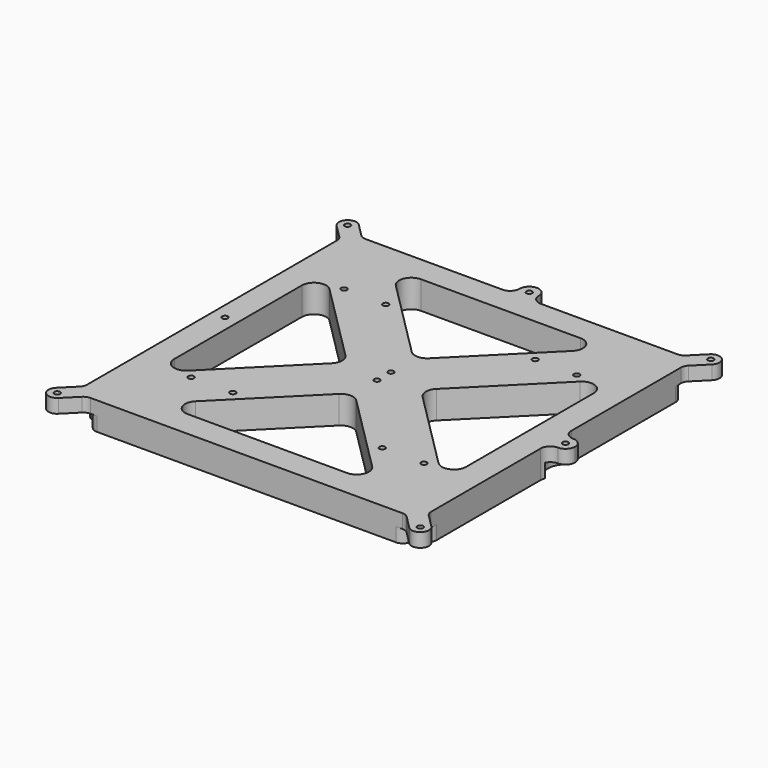
from build123d import *

# Parameters (mm, degrees)
F0_W         = 198
F0_H         = 198
F1_DEPTH     = 16
F2_W         = 11
F2_H         = 11
F3_DEPTH     = 16
F5_DEPTH     = 8
F6_R         = 5
F7_R         = 7
F8_T1_DEPTH  = 35.5
F8_T3_DEPTH  = 8
F8_T8_DEPTH  = 35.5
F8_S11_R     = 10
F8_T12_DEPTH = 20
F8_T16_DEPTH = 35.5
F8_S19_R     = 10
F8_T20_DEPTH = 20
F8_T24_DEPTH = 35.5
F8_S27_R     = 10
F8_T28_DEPTH = 20
F8_T32_DEPTH = 35.5
F8_S35_R     = 10
F8_T36_DEPTH = 20
F9_D         = 3.3
F10_D        = 3.3
F11_D        = 3.3


# Not quite as in the source:
# - a fillet or chamfer that OpenCascade refuses, or shapes differently, is made with other operations: its cross-section is extruded or revolved along the edge and cut away or added
# - ends of sketch curves that miss each other by under 0.0002 mm in the source are joined


with BuildPart() as f1:
    # F0 (on Top) → F1 (new body)
    with BuildSketch(Plane.XY):
        Rectangle(F0_W, F0_H)
        Polygon((-62.7867965644, -84), (0, -21.2132034356), (62.7867965644, -84), align=None, mode=Mode.SUBTRACT)
        Polygon((84, -62.7867965644), (21.2132034356, 0), (84, 62.7867965644), align=None, mode=Mode.SUBTRACT)
        Polygon((-84, 62.7867965644), (-21.2132034356, 0), (-84, -62.7867965644), align=None, mode=Mode.SUBTRACT)
        Polygon((62.7867965644, 84), (0, 21.2132034356), (-62.7867965644, 84), align=None, mode=Mode.SUBTRACT)
    extrude(amount=F1_DEPTH)

    # F2 (on face) → F3 (join, through all)
    with BuildSketch(Plane.XY.offset(16)):
        with BuildLine():
            Line((-99, -99), (-99, -91.9289296269))
            Line((-99, -91.9289296269), (-108.0355351865, -100.9644648135))
            ThreePointArc((-108.0355351865, -100.9644648135), (-108.0355351865, -108.0355351865), (-100.9644648135, -108.0355351865))
            Line((-100.9644648135, -108.0355351865), (-91.9289321881, -99))
            Line((-91.9289321881, -99), (-99, -99))
        make_face()
        with BuildLine():
            Line((99, -99), (91.9289321881, -99))
            Line((91.9289321881, -99), (100.9644660941, -108.0355339059))
            ThreePointArc((100.9644660941, -108.0355339059), (108.0355351865, -108.0355351865), (108.0355351865, -100.9644648135))
            Line((108.0355351865, -100.9644648135), (99, -91.9289296269))
            Line((99, -91.9289296269), (99, -99))
        make_face()
        with Locations((104.5, 0)):
            Rectangle(F2_W, F2_H)
        with BuildLine():
            Line((100.9644660941, 108.0355339059), (91.9289321881, 99))
            Line((91.9289321881, 99), (99, 99))
            Line((99, 99), (99, 91.9289296269))
            Line((99, 91.9289296269), (108.0355351865, 100.9644648135))
            ThreePointArc((108.0355351865, 100.9644648135), (108.0355351865, 108.0355351865), (100.9644660941, 108.0355339059))
        make_face()
        with BuildLine():
            Line((-99, 99), (-91.9289321881, 99))
            Line((-91.9289321881, 99), (-100.9644660941, 108.0355339059))
            ThreePointArc((-100.9644660941, 108.0355339059), (-108.0355351865, 108.0355351865), (-108.0355351865, 100.9644648135))
            Line((-108.0355351865, 100.9644648135), (-99, 91.9289296269))
            Line((-99, 91.9289296269), (-99, 99))
        make_face()
        with Locations((0, 104.5)):
            Rectangle(F2_W, F2_H)
    extrude(amount=-F3_DEPTH)

    # F4 (on face) → F5 (cut)
    with BuildSketch(Plane(origin=(0, 0, 0), x_dir=(1, 0, 0), z_dir=(0, 0, -1))):
        with BuildLine():
            Line((-99, 91.9289296269), (-99, 89.5562516017))
            ThreePointArc((-99, 89.5562516017), (-92.9111652352, 92.9111652352), (-89.5562516017, 99))
            Line((-89.5562516017, 99), (-91.9289321881, 99))
            Line((-91.9289321881, 99), (-100.9644648135, 108.0355351865))
            ThreePointArc((-100.9644648135, 108.0355351865), (-108.0355351865, 108.0355351865), (-108.0355351865, 100.9644648135))
            Line((-108.0355351865, 100.9644648135), (-99, 91.9289296269))
        make_face()
        with BuildLine():
            Line((91.9289321881, 99), (89.5562516017, 99))
            ThreePointArc((89.5562516017, 99), (92.9111652352, 92.9111652352), (99, 89.5562516017))
            Line((99, 89.5562516017), (99, 91.9289296269))
            Line((99, 91.9289296269), (108.0355351865, 100.9644648135))
            ThreePointArc((108.0355351865, 100.9644648135), (108.0355358268, 108.0355345462), (100.9644660941, 108.0355339059))
            Line((100.9644660941, 108.0355339059), (91.9289321881, 99))
        make_face()
        with BuildLine():
            ThreePointArc((-89.5562516017, -99), (-92.9111652352, -92.9111652352), (-99, -89.5562516017))
            Line((-99, -89.5562516017), (-99, -91.9289296269))
            Line((-99, -91.9289296269), (-108.0355351865, -100.9644648135))
            ThreePointArc((-108.0355351865, -100.9644648135), (-108.0355358268, -108.0355345462), (-100.9644660941, -108.0355339059))
            Line((-100.9644660941, -108.0355339059), (-91.9289321881, -99))
            Line((-91.9289321881, -99), (-89.5562516017, -99))
        make_face()
        with BuildLine():
            Line((99, 5.5), (99, 8.3516465442))
            ThreePointArc((99, 8.3516465442), (94.5, 0), (99, -8.3516465442))
            Line((99, -8.3516465442), (99, -5.5))
            Line((99, -5.5), (110, -5.5))
            Line((110, -5.5), (110, 5.5))
            Line((110, 5.5), (99, 5.5))
        make_face()
        with BuildLine():
            ThreePointArc((114.5, 0), (109.2434164903, 8.8034084308), (99, 8.3516465442))
            Line((99, 8.3516465442), (99, 5.5))
            Line((99, 5.5), (110, 5.5))
            Line((110, 5.5), (110, -5.5))
            Line((110, -5.5), (99, -5.5))
            Line((99, -5.5), (99, -8.3516465442))
            ThreePointArc((99, -8.3516465442), (109.2434164903, -8.8034084308), (114.5, 0))
        make_face()
        with BuildLine():
            Line((-5.5, -99), (-8.3516465442, -99))
            ThreePointArc((-8.3516465442, -99), (-2.8708478327, -114.0790517652), (10, -104.5))
            ThreePointArc((10, -104.5), (9.5790517652, -101.6291521673), (8.3516465442, -99))
            Line((8.3516465442, -99), (5.5, -99))
            Line((5.5, -99), (5.5, -110))
            Line((5.5, -110), (-5.5, -110))
            Line((-5.5, -110), (-5.5, -99))
        make_face()
        with BuildLine():
            ThreePointArc((8.3516465442, -99), (0, -94.5), (-8.3516465442, -99))
            Line((-8.3516465442, -99), (-5.5, -99))
            Line((-5.5, -99), (-5.5, -110))
            Line((-5.5, -110), (5.5, -110))
            Line((5.5, -110), (5.5, -99))
            Line((5.5, -99), (8.3516465442, -99))
        make_face()
        with BuildLine():
            Line((99, -91.9289296269), (99, -89.5562516017))
            ThreePointArc((99, -89.5562516017), (92.9111652352, -92.9111652352), (89.5562516017, -99))
            Line((89.5562516017, -99), (91.9289321881, -99))
            Line((91.9289321881, -99), (100.9644660941, -108.0355339059))
            ThreePointArc((100.9644660941, -108.0355339059), (108.0355358268, -108.0355345462), (108.0355351865, -100.9644648135))
            Line((108.0355351865, -100.9644648135), (99, -91.9289296269))
        make_face()
    extrude(amount=-F5_DEPTH, mode=Mode.SUBTRACT)

    # F6
    f6_edges = [f1.edges().sort_by_distance(p)[0] for p in [
        (-91.928932, 99, 12),
        (-99, 91.92893, 12),
        (-99, -91.92893, 12),
        (-91.928932, -99, 12),
        (91.928932, -99, 12),
        (99, -91.92893, 12),
        (99, 91.92893, 12),
        (91.928932, 99, 12),
        (89.556252, 99, 4),
        (99, 89.556252, 4),
        (99, -89.556252, 4),
        (89.556252, -99, 4),
        (-89.556252, -99, 4),
        (-99, -89.556252, 4),
        (-89.556252, 99, 4),
        (-99, 89.556252, 4),
    ]]
    fillet(f6_edges, radius=F6_R)

    # F7
    f7_edges = [f1.edges().sort_by_distance(p)[0] for p in [
        (-84, -62.786797, 8),
        (-84, 62.786797, 8),
        (-21.213203, 0, 8),
        (62.786797, -84, 8),
        (-62.786797, -84, 8),
        (0, -21.213203, 8),
        (21.213203, 0, 8),
        (84, -62.786797, 8),
        (84, 62.786797, 8),
        (62.786797, 84, 8),
        (0, 21.213203, 8),
        (-62.786797, 84, 8),
    ]]
    fillet(f7_edges, radius=F7_R)

    # F8: fillet of radius 5.5 on 8 edges, made by hand

    # F8_s2 → F8_t1 (cut)
    with BuildSketch(Plane.XY.offset(-5.75)):
        with BuildLine():
            ThreePointArc((104.5, -5.5), (108.3890872965, -3.8890872965), (110, 0))
            Line((110, 0), (110, -5.5))
            Line((110, -5.5), (104.5, -5.5))
        make_face()
        with BuildLine():
            ThreePointArc((104.5, 5.5), (108.3890872965, 3.8890872965), (110, 0))
            Line((110, 0), (110, 5.5))
            Line((110, 5.5), (104.5, 5.5))
        make_face()
        with BuildLine():
            ThreePointArc((-5.5, 104.5), (-3.8890872965, 108.3890872965), (0, 110))
            Line((0, 110), (-5.5, 110))
            Line((-5.5, 110), (-5.5, 104.5))
        make_face()
        with BuildLine():
            ThreePointArc((5.5, 104.5), (3.8890872965, 108.3890872965), (0, 110))
            Line((0, 110), (5.5, 110))
            Line((5.5, 110), (5.5, 104.5))
        make_face()
    extrude(amount=F8_T1_DEPTH, mode=Mode.SUBTRACT)

    # F8_s4 → F8_t3 (join)
    with BuildSketch(Plane.XY.offset(8)):
        with BuildLine():
            ThreePointArc((104.5, -5.5), (100.6109127035, -7.1109127035), (99, -11))
            Line((99, -11), (99, -5.5))
            Line((99, -5.5), (104.5, -5.5))
        make_face()
        with BuildLine():
            ThreePointArc((104.5, 5.5), (100.6109127035, 7.1109127035), (99, 11))
            Line((99, 11), (99, 5.5))
            Line((99, 5.5), (104.5, 5.5))
        make_face()
        with BuildLine():
            ThreePointArc((-5.5, 104.5), (-7.1109127035, 100.6109127035), (-11, 99))
            Line((-11, 99), (-5.5, 99))
            Line((-5.5, 99), (-5.5, 104.5))
        make_face()
        with BuildLine():
            ThreePointArc((5.5, 104.5), (7.1109127035, 100.6109127035), (11, 99))
            Line((11, 99), (5.5, 99))
            Line((5.5, 99), (5.5, 104.5))
        make_face()
    extrude(amount=F8_T3_DEPTH)


with BuildPart() as f8_tool6:
    # F8_s7 → F8_t8 (new body)
    with BuildSketch(Plane.XY.offset(29.75)):
        with BuildLine():
            ThreePointArc((104.5, -5.5), (100.6109127035, -7.1109127035), (99, -11))
            Line((99, -11), (99, -5.5))
            Line((99, -5.5), (104.5, -5.5))
        make_face()
    extrude(amount=-F8_T8_DEPTH)

    split(bisect_by=Plane.XY, keep=Keep.TOP)

    split(bisect_by=Plane.XY.offset(8), keep=Keep.BOTTOM)

    # F8_s11 → F8_t12 (cut, symmetric)
    with BuildSketch(Plane.XY.offset(12)):
        with Locations((104.5, 0)):
            Circle(F8_S11_R)
    extrude(amount=F8_T12_DEPTH, both=True, mode=Mode.SUBTRACT)


with BuildPart() as f1_1:
    add(f1.part)

    # F8_t5: union F8_tool6
    add(f8_tool6.part)


with BuildPart() as f8_tool14:
    # F8_s15 → F8_t16 (new body)
    with BuildSketch(Plane.XY.offset(29.75)):
        with BuildLine():
            ThreePointArc((104.5, 5.5), (100.6109127035, 7.1109127035), (99, 11))
            Line((99, 11), (99, 5.5))
            Line((99, 5.5), (104.5, 5.5))
        make_face()
    extrude(amount=-F8_T16_DEPTH)

    split(bisect_by=Plane.XY, keep=Keep.TOP)

    split(bisect_by=Plane.XY.offset(8), keep=Keep.BOTTOM)

    # F8_s19 → F8_t20 (cut, symmetric)
    with BuildSketch(Plane.XY.offset(12)):
        with Locations((104.5, 0)):
            Circle(F8_S19_R)
    extrude(amount=F8_T20_DEPTH, both=True, mode=Mode.SUBTRACT)


with BuildPart() as f1_2:
    add(f1_1.part)

    # F8_t13: union F8_tool14
    add(f8_tool14.part)


with BuildPart() as f8_tool22:
    # F8_s23 → F8_t24 (new body)
    with BuildSketch(Plane.XY.offset(29.75)):
        with BuildLine():
            ThreePointArc((-5.5, 104.5), (-7.1109127035, 100.6109127035), (-11, 99))
            Line((-11, 99), (-5.5, 99))
            Line((-5.5, 99), (-5.5, 104.5))
        make_face()
    extrude(amount=-F8_T24_DEPTH)

    split(bisect_by=Plane.XY, keep=Keep.TOP)

    split(bisect_by=Plane.XY.offset(8), keep=Keep.BOTTOM)

    # F8_s27 → F8_t28 (cut, symmetric)
    with BuildSketch(Plane.XY.offset(12)):
        with Locations((0, 104.5)):
            Circle(F8_S27_R)
    extrude(amount=F8_T28_DEPTH, both=True, mode=Mode.SUBTRACT)


with BuildPart() as f1_3:
    add(f1_2.part)

    # F8_t21: union F8_tool22
    add(f8_tool22.part)


with BuildPart() as f8_tool30:
    # F8_s31 → F8_t32 (new body)
    with BuildSketch(Plane.XY.offset(29.75)):
        with BuildLine():
            ThreePointArc((5.5, 104.5), (7.1109127035, 100.6109127035), (11, 99))
            Line((11, 99), (5.5, 99))
            Line((5.5, 99), (5.5, 104.5))
        make_face()
    extrude(amount=-F8_T32_DEPTH)

    split(bisect_by=Plane.XY, keep=Keep.TOP)

    split(bisect_by=Plane.XY.offset(8), keep=Keep.BOTTOM)

    # F8_s35 → F8_t36 (cut, symmetric)
    with BuildSketch(Plane.XY.offset(12)):
        with Locations((0, 104.5)):
            Circle(F8_S35_R)
    extrude(amount=F8_T36_DEPTH, both=True, mode=Mode.SUBTRACT)


with BuildPart() as f1_4:
    add(f1_3.part)

    # F8_t29: union F8_tool30
    add(f8_tool30.part)

    # F9 (through all)
    with Locations(Plane.XY.offset(16)):
        with Locations((104.5, 104.5), (-104.5, 104.5), (-104.5, -104.5), (104.5, -104.5), (0, -5), (0, 5), (0, 104.5), (104.5, 0)):
            Hole(F9_D / 2)

    # F10 (through all)
    with Locations(Plane(origin=(0, 0, 0), x_dir=(1, 0, 0), z_dir=(0, 0, -1))):
        with Locations((67, 55), (43, 55), (-43, 55), (-67, 55), (-67, -55), (-43, -55), (43, -55), (67, -55)):
            Hole(F10_D / 2)

    # F11 (through all)
    with Locations(Plane(origin=(0, 0, 0), x_dir=(1, 0, 0), z_dir=(0, 0, -1))):
        with Locations((-91.5, 0)):
            Hole(F11_D / 2)


solid = f1_4.part
